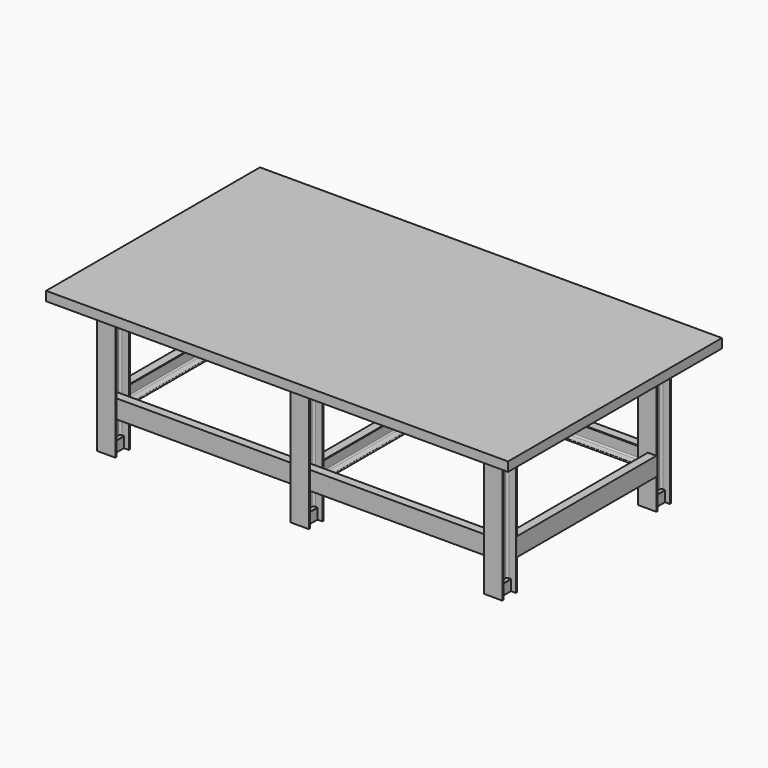
from build123d import *

# Parameters (mm, degrees)
F1_DEPTH  = 800
F3_W      = 60
F3_H      = 98
F4_DEPTH  = 70
F5_W      = 120
F5_H      = 11
F6_DEPTH  = 70
F7_R      = 8
F8_DEPTH  = 70
F9_SIZE   = 1
F9_2_SIZE = 1
F9_3_SIZE = 1
F9_4_SIZE = 1
F9_5_SIZE = 1
F9_6_SIZE = 1
F11_DEPTH = 1250
F13_DEPTH = 1250
F15_DEPTH = 1130
F16_W     = 3000
F16_H     = 1736
F17_DEPTH = 60


with BuildPart() as f1:
    # F0 (on Top) → F1 (new body)
    with BuildSketch(Plane.XY):
        with BuildLine():
            Line((60, 60), (0, 60))
            Line((0, 60), (-60, 60))
            Line((-60, 60), (-60, 49))
            Line((-60, 49), (-15.75, 49))
            ThreePointArc((-15.75, 49), (-6.9111652352, 45.3388347648), (-3.25, 36.5))
            Line((-3.25, 36.5), (-3.25, -36.5))
            ThreePointArc((-3.25, -36.5), (-6.9111652352, -45.3388347648), (-15.75, -49))
            Line((-15.75, -49), (-60, -49))
            Line((-60, -49), (-60, -60))
            Line((-60, -60), (0, -60))
            Line((0, -60), (60, -60))
            Line((60, -60), (60, -49))
            Line((60, -49), (15.75, -49))
            ThreePointArc((15.75, -49), (6.9111652352, -45.3388347648), (3.25, -36.5))
            Line((3.25, -36.5), (3.25, 36.5))
            ThreePointArc((3.25, 36.5), (6.9111652352, 45.3388347648), (15.75, 49))
            Line((15.75, 49), (60, 49))
            Line((60, 49), (60, 60))
        make_face()
    extrude(amount=F1_DEPTH)

    # F5 (on face) → F6 (join)
    with BuildSketch(Plane(origin=(0, 0, 0), x_dir=(1, 0, 0), z_dir=(0, 0, -1))):
        with Locations((0, -54.5)):
            Rectangle(F5_W, F5_H)
        with Locations((0, 54.5)):
            Rectangle(F5_W, F5_H)
    extrude(amount=F6_DEPTH)


with BuildPart() as f1b:
    # F0 (on Top) → F1, piece 2 (new body)
    with BuildSketch(Plane.XY):
        with BuildLine():
            ThreePointArc((-1253.25, 36.5), (-1249.5888347648, 45.3388347648), (-1240.75, 49))
            Line((-1240.75, 49), (-1196.5, 49))
            Line((-1196.5, 49), (-1196.5, 60))
            Line((-1196.5, 60), (-1256.5, 60))
            Line((-1256.5, 60), (-1316.5, 60))
            Line((-1316.5, 60), (-1316.5, 49))
            Line((-1316.5, 49), (-1272.25, 49))
            ThreePointArc((-1272.25, 49), (-1263.4111652352, 45.3388347648), (-1259.75, 36.5))
            Line((-1259.75, 36.5), (-1259.75, -36.5))
            ThreePointArc((-1259.75, -36.5), (-1263.4111652352, -45.3388347648), (-1272.25, -49))
            Line((-1272.25, -49), (-1316.5, -49))
            Line((-1316.5, -49), (-1316.5, -60))
            Line((-1316.5, -60), (-1256.5, -60))
            Line((-1256.5, -60), (-1196.5, -60))
            Line((-1196.5, -60), (-1196.5, -49))
            Line((-1196.5, -49), (-1240.75, -49))
            ThreePointArc((-1240.75, -49), (-1249.5888347648, -45.3388347648), (-1253.25, -36.5))
            Line((-1253.25, -36.5), (-1253.25, 36.5))
        make_face()
    extrude(amount=F1_DEPTH)

    # F5 (on face) → F6, piece 2 (join)
    with BuildSketch(Plane(origin=(0, 0, 0), x_dir=(1, 0, 0), z_dir=(0, 0, -1))):
        with Locations((-1256.5, 54.5)):
            Rectangle(F5_W, F5_H)
        with Locations((-1256.5, -54.5)):
            Rectangle(F5_W, F5_H)
    extrude(amount=F6_DEPTH)


with BuildPart() as f1c:
    # F0 (on Top) → F1, piece 3 (new body)
    with BuildSketch(Plane.XY):
        with BuildLine():
            Line((-2516.25, 36.5), (-2516.25, -36.5))
            ThreePointArc((-2516.25, -36.5), (-2519.9111652352, -45.3388347648), (-2528.75, -49))
            Line((-2528.75, -49), (-2573, -49))
            Line((-2573, -49), (-2573, -60))
            Line((-2573, -60), (-2513, -60))
            Line((-2513, -60), (-2453, -60))
            Line((-2453, -60), (-2453, -49))
            Line((-2453, -49), (-2497.25, -49))
            ThreePointArc((-2497.25, -49), (-2506.0888347648, -45.3388347648), (-2509.75, -36.5))
            Line((-2509.75, -36.5), (-2509.75, 36.5))
            ThreePointArc((-2509.75, 36.5), (-2506.0888347648, 45.3388347648), (-2497.25, 49))
            Line((-2497.25, 49), (-2453, 49))
            Line((-2453, 49), (-2453, 60))
            Line((-2453, 60), (-2513, 60))
            Line((-2513, 60), (-2573, 60))
            Line((-2573, 60), (-2573, 49))
            Line((-2573, 49), (-2528.75, 49))
            ThreePointArc((-2528.75, 49), (-2519.9111652352, 45.3388347648), (-2516.25, 36.5))
        make_face()
    extrude(amount=F1_DEPTH)

    # F5 (on face) → F6, piece 3 (join)
    with BuildSketch(Plane(origin=(0, 0, 0), x_dir=(1, 0, 0), z_dir=(0, 0, -1))):
        with Locations((-2513, 54.5)):
            Rectangle(F5_W, F5_H)
        with Locations((-2513, -54.5)):
            Rectangle(F5_W, F5_H)
    extrude(amount=F6_DEPTH)


with BuildPart() as f1d:
    # F0 (on Top) → F1, piece 4 (new body)
    with BuildSketch(Plane.XY):
        with BuildLine():
            ThreePointArc((-1240.75, -1299), (-1249.5888347648, -1295.3388347648), (-1253.25, -1286.5))
            Line((-1253.25, -1286.5), (-1253.25, -1213.5))
            ThreePointArc((-1253.25, -1213.5), (-1249.5888347648, -1204.6611652352), (-1240.75, -1201))
            Line((-1240.75, -1201), (-1196.5, -1201))
            Line((-1196.5, -1201), (-1196.5, -1190))
            Line((-1196.5, -1190), (-1256.5, -1190))
            Line((-1256.5, -1190), (-1316.5, -1190))
            Line((-1316.5, -1190), (-1316.5, -1201))
            Line((-1316.5, -1201), (-1272.25, -1201))
            ThreePointArc((-1272.25, -1201), (-1263.4111652352, -1204.6611652352), (-1259.75, -1213.5))
            Line((-1259.75, -1213.5), (-1259.75, -1286.5))
            ThreePointArc((-1259.75, -1286.5), (-1263.4111652352, -1295.3388347648), (-1272.25, -1299))
            Line((-1272.25, -1299), (-1316.5, -1299))
            Line((-1316.5, -1299), (-1316.5, -1310))
            Line((-1316.5, -1310), (-1256.5, -1310))
            Line((-1256.5, -1310), (-1196.5, -1310))
            Line((-1196.5, -1310), (-1196.5, -1299))
            Line((-1196.5, -1299), (-1240.75, -1299))
        make_face()
    extrude(amount=F1_DEPTH)

    # F5 (on face) → F6, piece 6 (join)
    with BuildSketch(Plane(origin=(0, 0, 0), x_dir=(1, 0, 0), z_dir=(0, 0, -1))):
        with Locations((-1256.5, 1304.5)):
            Rectangle(F5_W, F5_H)
        with Locations((-1256.5, 1195.5)):
            Rectangle(F5_W, F5_H)
    extrude(amount=F6_DEPTH)


with BuildPart() as f1e:
    # F0 (on Top) → F1, piece 5 (new body)
    with BuildSketch(Plane.XY):
        with BuildLine():
            Line((60, -1299), (15.75, -1299))
            ThreePointArc((15.75, -1299), (6.9111652352, -1295.3388347648), (3.25, -1286.5))
            Line((3.25, -1286.5), (3.25, -1213.5))
            ThreePointArc((3.25, -1213.5), (6.9111652352, -1204.6611652352), (15.75, -1201))
            Line((15.75, -1201), (60, -1201))
            Line((60, -1201), (60, -1190))
            Line((60, -1190), (0, -1190))
            Line((0, -1190), (-60, -1190))
            Line((-60, -1190), (-60, -1201))
            Line((-60, -1201), (-15.75, -1201))
            ThreePointArc((-15.75, -1201), (-6.9111652352, -1204.6611652352), (-3.25, -1213.5))
            Line((-3.25, -1213.5), (-3.25, -1286.5))
            ThreePointArc((-3.25, -1286.5), (-6.9111652352, -1295.3388347648), (-15.75, -1299))
            Line((-15.75, -1299), (-60, -1299))
            Line((-60, -1299), (-60, -1310))
            Line((-60, -1310), (0, -1310))
            Line((0, -1310), (60, -1310))
            Line((60, -1310), (60, -1299))
        make_face()
    extrude(amount=F1_DEPTH)

    # F5 (on face) → F6, piece 5 (join)
    with BuildSketch(Plane(origin=(0, 0, 0), x_dir=(1, 0, 0), z_dir=(0, 0, -1))):
        with Locations((0, 1304.5)):
            Rectangle(F5_W, F5_H)
        with Locations((0, 1195.5)):
            Rectangle(F5_W, F5_H)
    extrude(amount=F6_DEPTH)


with BuildPart() as f1f:
    # F0 (on Top) → F1, piece 6 (new body)
    with BuildSketch(Plane.XY):
        with BuildLine():
            ThreePointArc((-2528.75, -1201), (-2519.9111652352, -1204.6611652352), (-2516.25, -1213.5))
            Line((-2516.25, -1213.5), (-2516.25, -1286.5))
            ThreePointArc((-2516.25, -1286.5), (-2519.9111652352, -1295.3388347648), (-2528.75, -1299))
            Line((-2528.75, -1299), (-2573, -1299))
            Line((-2573, -1299), (-2573, -1310))
            Line((-2573, -1310), (-2513, -1310))
            Line((-2513, -1310), (-2453, -1310))
            Line((-2453, -1310), (-2453, -1299))
            Line((-2453, -1299), (-2497.25, -1299))
            ThreePointArc((-2497.25, -1299), (-2506.0888347648, -1295.3388347648), (-2509.75, -1286.5))
            Line((-2509.75, -1286.5), (-2509.75, -1213.5))
            ThreePointArc((-2509.75, -1213.5), (-2506.0888347648, -1204.6611652352), (-2497.25, -1201))
            Line((-2497.25, -1201), (-2453, -1201))
            Line((-2453, -1201), (-2453, -1190))
            Line((-2453, -1190), (-2513, -1190))
            Line((-2513, -1190), (-2573, -1190))
            Line((-2573, -1190), (-2573, -1201))
            Line((-2573, -1201), (-2528.75, -1201))
        make_face()
    extrude(amount=F1_DEPTH)

    # F5 (on face) → F6, piece 4 (join)
    with BuildSketch(Plane(origin=(0, 0, 0), x_dir=(1, 0, 0), z_dir=(0, 0, -1))):
        with Locations((-2513, 1304.5)):
            Rectangle(F5_W, F5_H)
        with Locations((-2513, 1195.5)):
            Rectangle(F5_W, F5_H)
    extrude(amount=F6_DEPTH)


with BuildPart() as f4:
    # F3 (on face) → F4 (new body)
    with BuildSketch(Plane(origin=(0, 0, 0), x_dir=(1, 0, 0), z_dir=(0, 0, -1))):
        Rectangle(F3_W, F3_H)
    extrude(amount=F4_DEPTH)


with BuildPart() as f4b:
    # F3 (on face) → F4, piece 2 (new body)
    with BuildSketch(Plane(origin=(0, 0, 0), x_dir=(1, 0, 0), z_dir=(0, 0, -1))):
        with Locations((-1256.5, 0)):
            Rectangle(F3_W, F3_H)
    extrude(amount=F4_DEPTH)


with BuildPart() as f4c:
    # F3 (on face) → F4, piece 3 (new body)
    with BuildSketch(Plane(origin=(0, 0, 0), x_dir=(1, 0, 0), z_dir=(0, 0, -1))):
        with Locations((-2513, 0)):
            Rectangle(F3_W, F3_H)
    extrude(amount=F4_DEPTH)


with BuildPart() as f4d:
    # F3 (on face) → F4, piece 4 (new body)
    with BuildSketch(Plane(origin=(0, 0, 0), x_dir=(1, 0, 0), z_dir=(0, 0, -1))):
        with Locations((-2513, 1250)):
            Rectangle(F3_W, F3_H)
    extrude(amount=F4_DEPTH)


with BuildPart() as f4e:
    # F3 (on face) → F4, piece 5 (new body)
    with BuildSketch(Plane(origin=(0, 0, 0), x_dir=(1, 0, 0), z_dir=(0, 0, -1))):
        with Locations((-1256.5, 1250)):
            Rectangle(F3_W, F3_H)
    extrude(amount=F4_DEPTH)


with BuildPart() as f4f:
    # F3 (on face) → F4, piece 6 (new body)
    with BuildSketch(Plane(origin=(0, 0, 0), x_dir=(1, 0, 0), z_dir=(0, 0, -1))):
        with Locations((0, 1250)):
            Rectangle(F3_W, F3_H)
    extrude(amount=F4_DEPTH)


with BuildPart() as f8_tool:
    # F7 (on face) → F8 (new body)
    with BuildSketch(Plane(origin=(0, 0, -70), x_dir=(1, 0, 0), z_dir=(0, 0, -1))):
        Circle(F7_R)
        with Locations((0, 1250)):
            Circle(F7_R)
        with Locations((-1256.5, 1250)):
            Circle(F7_R)
        with Locations((-2513, 1250)):
            Circle(F7_R)
        with Locations((-2513, 0)):
            Circle(F7_R)
        with Locations((-1256.5, 0)):
            Circle(F7_R)
    extrude(amount=-F8_DEPTH)


with BuildPart() as f4_1:
    add(f4.part)

    # F8: cut by f8_tool
    add(f8_tool.part, mode=Mode.SUBTRACT)

    # F9
    f9_edges = [f4_1.edges().sort_by_distance(p)[0] for p in [
        (30, 0, 0),
        (30, 0, -70),
        (-30, 0, -70),
        (-30, 0, 0),
    ]]
    chamfer(f9_edges, length=F9_SIZE)


with BuildPart() as f4b_1:
    add(f4b.part)

    # F8: cut by f8_tool
    add(f8_tool.part, mode=Mode.SUBTRACT)

    # F9#2
    f9_2_edges = [f4b_1.edges().sort_by_distance(p)[0] for p in [
        (-1226.5, 0, 0),
        (-1226.5, 0, -70),
        (-1286.5, 0, -70),
        (-1286.5, 0, 0),
    ]]
    chamfer(f9_2_edges, length=F9_2_SIZE)


with BuildPart() as f4c_1:
    add(f4c.part)

    # F8: cut by f8_tool
    add(f8_tool.part, mode=Mode.SUBTRACT)

    # F9#3
    f9_3_edges = [f4c_1.edges().sort_by_distance(p)[0] for p in [
        (-2543, 0, 0),
        (-2543, 0, -70),
        (-2483, 0, -70),
        (-2483, 0, 0),
    ]]
    chamfer(f9_3_edges, length=F9_3_SIZE)


with BuildPart() as f4d_1:
    add(f4d.part)

    # F8: cut by f8_tool
    add(f8_tool.part, mode=Mode.SUBTRACT)

    # F9#4
    f9_4_edges = [f4d_1.edges().sort_by_distance(p)[0] for p in [
        (-2483, -1250, 0),
        (-2483, -1250, -70),
        (-2543, -1250, -70),
        (-2543, -1250, 0),
    ]]
    chamfer(f9_4_edges, length=F9_4_SIZE)


with BuildPart() as f4e_1:
    add(f4e.part)

    # F8: cut by f8_tool
    add(f8_tool.part, mode=Mode.SUBTRACT)

    # F9#5
    f9_5_edges = [f4e_1.edges().sort_by_distance(p)[0] for p in [
        (-1286.5, -1250, 0),
        (-1286.5, -1250, -70),
        (-1226.5, -1250, -70),
        (-1226.5, -1250, 0),
    ]]
    chamfer(f9_5_edges, length=F9_5_SIZE)


with BuildPart() as f4f_1:
    add(f4f.part)

    # F8: cut by f8_tool
    add(f8_tool.part, mode=Mode.SUBTRACT)

    # F9#6
    f9_6_edges = [f4f_1.edges().sort_by_distance(p)[0] for p in [
        (30, -1250, 0),
        (30, -1250, -70),
        (-30, -1250, -70),
        (-30, -1250, 0),
    ]]
    chamfer(f9_6_edges, length=F9_6_SIZE)


with BuildPart() as f11:
    # F10 (on face) → F11 (new body, through all)
    with BuildSketch(Plane(origin=(-3.25, 0, 0), x_dir=(0, -1, 0), z_dir=(-1, 0, 0))):
        with BuildLine():
            Line((1277.5, 250), (1222.5, 250))
            Line((1222.5, 250), (1222.5, 247.4522430383))
            ThreePointArc((1222.5, 247.4522430383), (1223.6872369946, 244.4066558584), (1226.6224894535, 242.9681059098))
            Line((1226.6224894535, 242.9681059098), (1262.2550210931, 239.968274257))
            ThreePointArc((1262.2550210931, 239.968274257), (1268.1255260107, 237.0911743598), (1270.5, 231))
            Line((1270.5, 231), (1270.5, 190))
            Line((1270.5, 190), (1277.5, 190))
            Line((1277.5, 190), (1277.5, 250))
        make_face()
        with BuildLine():
            Line((1277.5, 130), (1277.5, 190))
            Line((1277.5, 190), (1270.5, 190))
            Line((1270.5, 190), (1270.5, 149))
            ThreePointArc((1270.5, 149), (1268.1255260107, 142.9088256402), (1262.2550210931, 140.031725743))
            Line((1262.2550210931, 140.031725743), (1226.6224894535, 137.0318940902))
            ThreePointArc((1226.6224894535, 137.0318940902), (1223.6872369946, 135.5933441416), (1222.5, 132.5477569617))
            Line((1222.5, 132.5477569617), (1222.5, 130))
            Line((1222.5, 130), (1277.5, 130))
        make_face()
    extrude(amount=F11_DEPTH)


with BuildPart() as f11b:
    # F10 (on face) → F11, piece 2 (new body, through all)
    with BuildSketch(Plane(origin=(-3.25, 0, 0), x_dir=(0, -1, 0), z_dir=(-1, 0, 0))):
        with BuildLine():
            Line((27.5, 247.4522430383), (27.5, 250))
            Line((27.5, 250), (-27.5, 250))
            Line((-27.5, 250), (-27.5, 190))
            Line((-27.5, 190), (-20.5, 190))
            Line((-20.5, 190), (-20.5, 231))
            ThreePointArc((-20.5, 231), (-18.1255260107, 237.0911743598), (-12.2550210931, 239.968274257))
            Line((-12.2550210931, 239.968274257), (23.3775105465, 242.9681059098))
            ThreePointArc((23.3775105465, 242.9681059098), (26.3127630054, 244.4066558584), (27.5, 247.4522430383))
        make_face()
        with BuildLine():
            Line((-20.5, 190), (-27.5, 190))
            Line((-27.5, 190), (-27.5, 130))
            Line((-27.5, 130), (27.5, 130))
            Line((27.5, 130), (27.5, 132.5477569617))
            ThreePointArc((27.5, 132.5477569617), (26.3127630054, 135.5933441416), (23.3775105465, 137.0318940902))
            Line((23.3775105465, 137.0318940902), (-12.2550210931, 140.031725743))
            ThreePointArc((-12.2550210931, 140.031725743), (-18.1255260107, 142.9088256402), (-20.5, 149))
            Line((-20.5, 149), (-20.5, 190))
        make_face()
    extrude(amount=F11_DEPTH)


with BuildPart() as f13:
    # F12 (on face) → F13 (new body, through all)
    with BuildSketch(Plane(origin=(-1259.75, 0, 0), x_dir=(0, -1, 0), z_dir=(-1, 0, 0))):
        with BuildLine():
            Line((1277.5, 250), (1222.5, 250))
            Line((1222.5, 250), (1222.5, 247.4522430383))
            ThreePointArc((1222.5, 247.4522430383), (1223.6872369946, 244.4066558584), (1226.6224894535, 242.9681059098))
            Line((1226.6224894535, 242.9681059098), (1262.2550210931, 239.968274257))
            ThreePointArc((1262.2550210931, 239.968274257), (1268.1255260107, 237.0911743598), (1270.5, 231))
            Line((1270.5, 231), (1270.5, 190))
            Line((1270.5, 190), (1270.5, 149))
            ThreePointArc((1270.5, 149), (1268.1255260107, 142.9088256402), (1262.2550210931, 140.031725743))
            Line((1262.2550210931, 140.031725743), (1226.6224894535, 137.0318940902))
            ThreePointArc((1226.6224894535, 137.0318940902), (1223.6872369946, 135.5933441416), (1222.5, 132.5477569617))
            Line((1222.5, 132.5477569617), (1222.5, 130))
            Line((1222.5, 130), (1277.5, 130))
            Line((1277.5, 130), (1277.5, 190))
            Line((1277.5, 190), (1277.5, 250))
        make_face()
    extrude(amount=F13_DEPTH)


with BuildPart() as f13b:
    # F12 (on face) → F13, piece 2 (new body, through all)
    with BuildSketch(Plane(origin=(-1259.75, 0, 0), x_dir=(0, -1, 0), z_dir=(-1, 0, 0))):
        with BuildLine():
            Line((27.5, 130), (27.5, 132.5477569617))
            ThreePointArc((27.5, 132.5477569617), (26.3127630054, 135.5933441416), (23.3775105465, 137.0318940902))
            Line((23.3775105465, 137.0318940902), (-12.2550210931, 140.031725743))
            ThreePointArc((-12.2550210931, 140.031725743), (-18.1255260107, 142.9088256402), (-20.5, 149))
            Line((-20.5, 149), (-20.5, 190))
            Line((-20.5, 190), (-20.5, 231))
            ThreePointArc((-20.5, 231), (-18.1255260107, 237.0911743598), (-12.2550210931, 239.968274257))
            Line((-12.2550210931, 239.968274257), (23.3775105465, 242.9681059098))
            ThreePointArc((23.3775105465, 242.9681059098), (26.3127630054, 244.4066558584), (27.5, 247.4522430383))
            Line((27.5, 247.4522430383), (27.5, 250))
            Line((27.5, 250), (-27.5, 250))
            Line((-27.5, 250), (-27.5, 190))
            Line((-27.5, 190), (-27.5, 130))
            Line((-27.5, 130), (27.5, 130))
        make_face()
    extrude(amount=F13_DEPTH)


with BuildPart() as f15:
    # F14 (on face) → F15 (new body, through all)
    with BuildSketch(Plane.XZ.offset(60)):
        with BuildLine():
            Line((-2518, 247.4522430383), (-2518, 250))
            Line((-2518, 250), (-2573, 250))
            Line((-2573, 250), (-2573, 190))
            Line((-2573, 190), (-2573, 130))
            Line((-2573, 130), (-2518, 130))
            Line((-2518, 130), (-2518, 132.5477569617))
            ThreePointArc((-2518, 132.5477569617), (-2519.1872369946, 135.5933441416), (-2522.1224894535, 137.0318940902))
            Line((-2522.1224894535, 137.0318940902), (-2557.7550210931, 140.031725743))
            ThreePointArc((-2557.7550210931, 140.031725743), (-2563.6255260107, 142.9088256402), (-2566, 149))
            Line((-2566, 149), (-2566, 190))
            Line((-2566, 190), (-2566, 231))
            ThreePointArc((-2566, 231), (-2563.6255260107, 237.0911743598), (-2557.7550210931, 239.968274257))
            Line((-2557.7550210931, 239.968274257), (-2522.1224894535, 242.9681059098))
            ThreePointArc((-2522.1224894535, 242.9681059098), (-2519.1872369946, 244.4066558584), (-2518, 247.4522430383))
        make_face()
    extrude(amount=F15_DEPTH)


with BuildPart() as f15b:
    # F14 (on face) → F15, piece 2 (new body, through all)
    with BuildSketch(Plane.XZ.offset(60)):
        with BuildLine():
            Line((9.1224894535, 242.9681059098), (44.7550210931, 239.968274257))
            ThreePointArc((44.7550210931, 239.968274257), (50.6255260107, 237.0911743598), (53, 231))
            Line((53, 231), (53, 190))
            Line((53, 190), (53, 149))
            ThreePointArc((53, 149), (50.6255260107, 142.9088256402), (44.7550210931, 140.031725743))
            Line((44.7550210931, 140.031725743), (9.1224894535, 137.0318940902))
            ThreePointArc((9.1224894535, 137.0318940902), (6.1872369946, 135.5933441416), (5, 132.5477569617))
            Line((5, 132.5477569617), (5, 130))
            Line((5, 130), (60, 130))
            Line((60, 130), (60, 190))
            Line((60, 190), (60, 250))
            Line((60, 250), (5, 250))
            Line((5, 250), (5, 247.4522430383))
            ThreePointArc((5, 247.4522430383), (6.1872369946, 244.4066558584), (9.1224894535, 242.9681059098))
        make_face()
    extrude(amount=F15_DEPTH)


with BuildPart() as f15c:
    # F14 (on face) → F15, piece 3 (new body, through all)
    with BuildSketch(Plane.XZ.offset(60)):
        with BuildLine():
            Line((-1229, 251), (-1284, 251))
            Line((-1284, 251), (-1284, 191))
            Line((-1284, 191), (-1284, 131))
            Line((-1284, 131), (-1229, 131))
            Line((-1229, 131), (-1229, 133.5477569617))
            ThreePointArc((-1229, 133.5477569617), (-1230.1872369946, 136.5933441416), (-1233.1224894535, 138.0318940902))
            Line((-1233.1224894535, 138.0318940902), (-1268.7550210931, 141.031725743))
            ThreePointArc((-1268.7550210931, 141.031725743), (-1274.6255260107, 143.9088256402), (-1277, 150))
            Line((-1277, 150), (-1277, 191))
            Line((-1277, 191), (-1277, 232))
            ThreePointArc((-1277, 232), (-1274.6255260107, 238.0911743598), (-1268.7550210931, 240.968274257))
            Line((-1268.7550210931, 240.968274257), (-1233.1224894535, 243.9681059098))
            ThreePointArc((-1233.1224894535, 243.9681059098), (-1230.1872369946, 245.4066558584), (-1229, 248.4522430383))
            Line((-1229, 248.4522430383), (-1229, 251))
        make_face()
    extrude(amount=F15_DEPTH)


with BuildPart() as f17:
    # F16 (on face) → F17 (new body)
    with BuildSketch(Plane.XY.offset(800)):
        with Locations((-1256.5, -625)):
            Rectangle(F16_W, F16_H)
    extrude(amount=F17_DEPTH)


solid = Compound([f1.part, f1b.part, f1c.part, f1d.part, f1e.part, f1f.part, f4_1.part, f4b_1.part, f4c_1.part, f4d_1.part, f4e_1.part, f4f_1.part, f11.part, f11b.part, f13.part, f13b.part, f15.part, f15b.part, f15c.part, f17.part])
